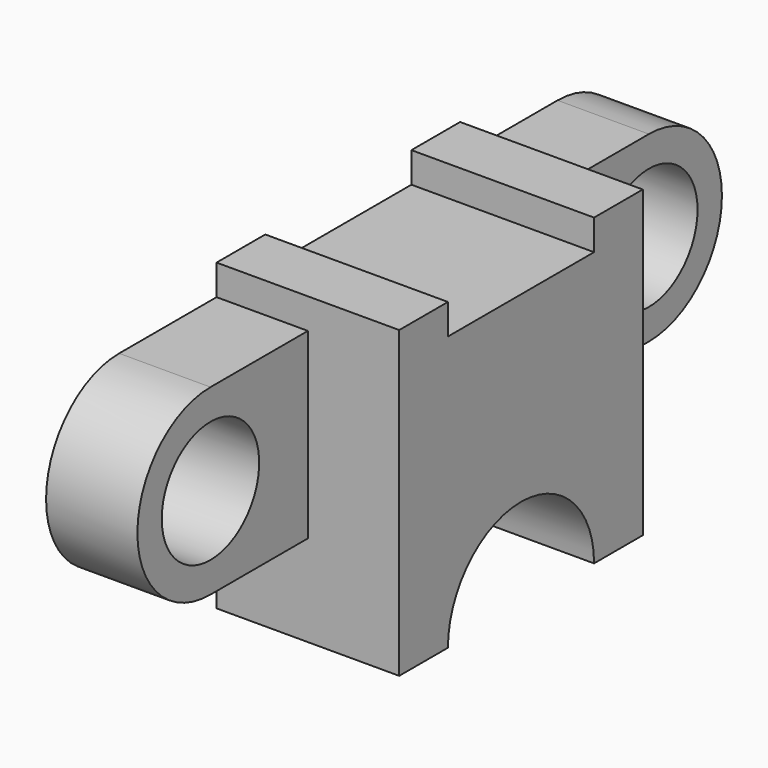
from build123d import *

# Parameters (mm, degrees)
F0_W     = 50
F0_H     = 50
F1_DEPTH = 30
F2_W     = 30
F2_H     = 5
F2_R     = 15
F3_DEPTH = 30.001
F4_R     = 10
F5_DEPTH = 15


# Not quite as in the source:
# - a pattern or mirror of a feature is missing from the dataset's text; its kind, count and spacing are read off the source's solid


with BuildPart() as f1:
    # F0 (on Right) → F1 (new body)
    with BuildSketch(Plane.YZ):
        Rectangle(F0_W, F0_H)
    extrude(amount=-F1_DEPTH)

    # F2 (on face) → F3 (cut, through all)
    with BuildSketch(Plane.YZ):
        with Locations((0, 22.5)):
            Rectangle(F2_W, F2_H)
        with Locations((0, -25)):
            Circle(F2_R)
    extrude(amount=-F3_DEPTH, mode=Mode.SUBTRACT)

    # F4 (on face) → F5 (join)
    with BuildSketch(Plane(origin=(-30, 0, 0), x_dir=(0, -1, 0), z_dir=(-1, 0, 0))):
        with BuildLine():
            Line((45, 20), (25, 20))
            Line((25, 20), (25, -10))
            Line((25, -10), (45, -10))
            ThreePointArc((45, -10), (55.6066017178, -5.6066017178), (60, 5))
            ThreePointArc((60, 5), (55.6066017178, 15.6066017178), (45, 20))
        make_face()
        with Locations((45, 5)):
            Circle(F4_R, mode=Mode.SUBTRACT)
    f5 = extrude(amount=-F5_DEPTH)

    # F5_copies: F5 across plane
    add(f5.mirror(Plane.ZX))


solid = f1.part
